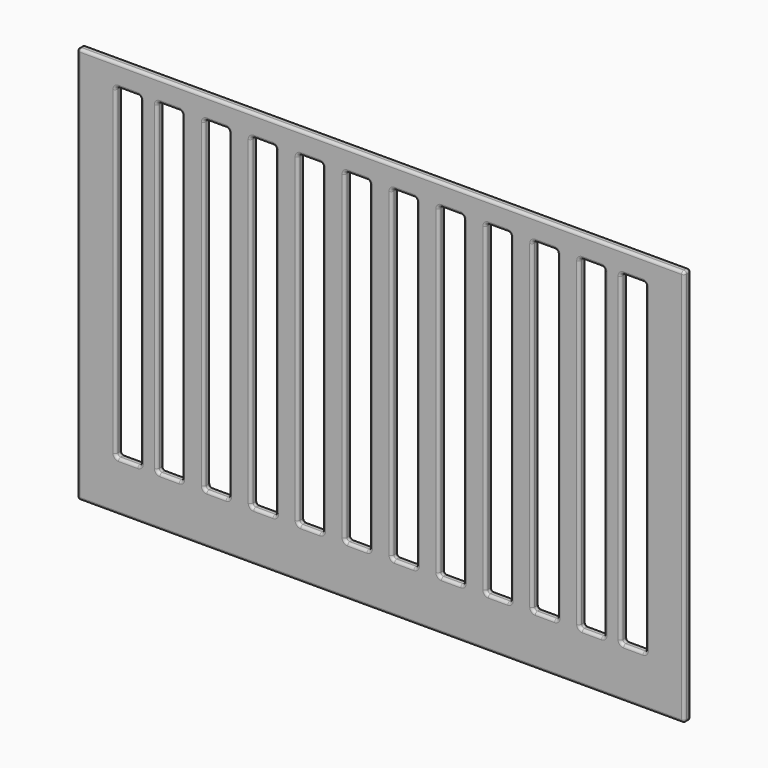
from build123d import *

# Parameters (mm, degrees)
F0_W     = 1397
F0_H     = 914.4
F1_DEPTH = 9.525
F2_W     = 57.15
F2_H     = 749.3
F3_DEPTH = 19.051
F4_F1_R  = 6.35
F4_F2_R  = 6.35
F4_F3_R  = 6.35


with BuildPart() as f1:
    # F0 (on Front) → F1 (new body, symmetric)
    with BuildSketch(Plane.XZ):
        Rectangle(F0_W, F0_H)
    extrude(amount=F1_DEPTH, both=True)

    # F2 (on face) → F3 (cut, through all)
    with BuildSketch(Plane.XZ.offset(9.525)):
        with Locations((-581.025, 31.75)):
            Rectangle(F2_W, F2_H)
        with Locations((-485.775, 31.75)):
            Rectangle(F2_W, F2_H)
        with Locations((-377.825, 31.75)):
            Rectangle(F2_W, F2_H)
        with Locations((-269.875, 31.75)):
            Rectangle(F2_W, F2_H)
        with Locations((-161.925, 31.75)):
            Rectangle(F2_W, F2_H)
        with Locations((-53.975, 31.75)):
            Rectangle(F2_W, F2_H)
        with Locations((53.975, 31.75)):
            Rectangle(F2_W, F2_H)
        with Locations((161.925, 31.75)):
            Rectangle(F2_W, F2_H)
        with Locations((269.875, 31.75)):
            Rectangle(F2_W, F2_H)
        with Locations((377.825, 31.75)):
            Rectangle(F2_W, F2_H)
        with Locations((485.775, 31.75)):
            Rectangle(F2_W, F2_H)
        with Locations((581.025, 31.75)):
            Rectangle(F2_W, F2_H)
    extrude(amount=-F3_DEPTH, mode=Mode.SUBTRACT)

    # F4: fillet of radius 6.35 on 135 edges, made by hand

    # F4_f1
    f4_f1_edges = [f1.edges().sort_by_distance(p)[0] for p in [
        (-82.55, 0, -342.9),
        (-82.55, 0, 406.4),
        (25.4, 0, -342.9),
        (25.4, 0, 406.4),
        (133.35, 0, -342.9),
        (133.35, 0, 406.4),
        (241.3, 0, -342.9),
        (241.3, 0, 406.4),
        (349.25, 0, -342.9),
        (349.25, 0, 406.4),
        (-190.5, 0, 406.4),
        (-298.45, 0, 406.4),
        (-241.3, 0, 406.4),
        (-406.4, 0, 406.4),
        (-349.25, 0, 406.4),
        (-514.35, 0, 406.4),
        (-457.2, 0, 406.4),
        (-609.6, 0, 406.4),
        (-552.45, 0, 406.4),
        (457.2, 0, -342.9),
        (457.2, 0, 406.4),
        (552.45, 0, -342.9),
        (552.45, 0, 406.4),
        (-552.45, 0, -342.9),
        (-609.6, 0, -342.9),
        (-457.2, 0, -342.9),
        (-514.35, 0, -342.9),
        (-349.25, 0, -342.9),
        (-406.4, 0, -342.9),
        (-241.3, 0, -342.9),
        (-298.45, 0, -342.9),
        (-133.35, 0, -342.9),
        (-190.5, 0, -342.9),
        (-25.4, 0, -342.9),
        (82.55, 0, -342.9),
        (190.5, 0, -342.9),
        (406.4, 0, -342.9),
        (514.35, 0, -342.9),
        (609.6, 0, -342.9),
        (609.6, 0, 406.4),
        (514.35, 0, 406.4),
        (406.4, 0, 406.4),
        (298.45, 0, 406.4),
        (298.45, 0, -342.9),
        (190.5, 0, 406.4),
        (82.55, 0, 406.4),
        (-25.4, 0, 406.4),
        (-133.35, 0, 406.4),
    ]]
    fillet(f4_f1_edges, radius=F4_F1_R)

    # F4_f2
    f4_f2_edges = [f1.edges().sort_by_distance(p)[0] for p in [
        (-698.5, -9.525, 0),
        (0, -9.525, 457.2),
        (0, 9.525, 457.2),
        (241.3, -9.525, 31.75),
        (241.3, 9.525, 31.75),
        (298.45, -9.525, 31.75),
        (698.5, 9.525, 0),
        (698.5, 0, 457.2),
        (698.5, -9.525, 0),
        (698.5, 0, -457.2),
        (-698.5, 0, 457.2),
        (-698.5, 9.525, 0),
        (-698.5, 0, -457.2),
        (0, 9.525, -457.2),
        (0, -9.525, -457.2),
        (298.45, 9.525, 31.75),
        (296.5901280605, 9.525, -341.0401280605),
        (296.5901280605, 9.525, 404.5401280605),
        (296.5901280605, -9.525, -341.0401280605),
        (296.5901280605, -9.525, 404.5401280605),
        (243.1598719395, 9.525, 404.5401280605),
        (243.1598719395, 9.525, -341.0401280605),
        (243.1598719395, -9.525, 404.5401280605),
        (243.1598719395, -9.525, -341.0401280605),
    ]]
    fillet(f4_f2_edges, radius=F4_F2_R)

    # F4_f3
    f4_f3_edges = [f1.edges().sort_by_distance(p)[0] for p in [
        (-609.6, -9.525, 31.75),
        (-609.6, 9.525, 31.75),
        (-552.45, -9.525, 31.75),
        (-514.35, -9.525, 31.75),
        (-514.35, 9.525, 31.75),
        (-457.2, -9.525, 31.75),
        (-406.4, -9.525, 31.75),
        (-406.4, 9.525, 31.75),
        (-349.25, -9.525, 31.75),
        (-298.45, -9.525, 31.75),
        (-298.45, 9.525, 31.75),
        (-241.3, -9.525, 31.75),
        (-269.875, -9.525, 406.4),
        (-377.825, -9.525, 406.4),
        (-485.775, -9.525, 406.4),
        (-581.025, -9.525, 406.4),
        (-161.925, -9.525, 406.4),
        (-190.5, -9.525, 31.75),
        (-190.5, 9.525, 31.75),
        (-133.35, -9.525, 31.75),
        (-82.55, -9.525, 31.75),
        (-82.55, 9.525, 31.75),
        (25.4, -9.525, 31.75),
        (25.4, 9.525, 31.75),
        (-25.4, -9.525, 31.75),
        (82.55, -9.525, 31.75),
        (133.35, -9.525, 31.75),
        (133.35, 9.525, 31.75),
        (190.5, -9.525, 31.75),
        (349.25, -9.525, 31.75),
        (349.25, 9.525, 31.75),
        (-269.875, 9.525, 406.4),
        (-377.825, 9.525, 406.4),
        (-485.775, 9.525, 406.4),
        (-581.025, 9.525, 406.4),
        (457.2, -9.525, 31.75),
        (457.2, 9.525, 31.75),
        (552.45, -9.525, 31.75),
        (552.45, 9.525, 31.75),
        (-581.025, -9.525, -342.9),
        (-581.025, 9.525, -342.9),
        (-485.775, -9.525, -342.9),
        (-485.775, 9.525, -342.9),
        (-377.825, -9.525, -342.9),
        (-377.825, 9.525, -342.9),
        (-269.875, -9.525, -342.9),
        (-269.875, 9.525, -342.9),
        (-161.925, -9.525, -342.9),
        (-161.925, 9.525, -342.9),
        (-53.975, -9.525, -342.9),
        (-53.975, 9.525, -342.9),
        (53.975, -9.525, -342.9),
        (53.975, 9.525, -342.9),
        (161.925, -9.525, -342.9),
        (161.925, 9.525, -342.9),
        (377.825, -9.525, -342.9),
        (377.825, 9.525, -342.9),
        (485.775, -9.525, -342.9),
        (485.775, 9.525, -342.9),
        (581.025, -9.525, -342.9),
        (581.025, 9.525, -342.9),
        (581.025, -9.525, 406.4),
        (581.025, 9.525, 406.4),
        (514.35, -9.525, 31.75),
        (514.35, 9.525, 31.75),
        (406.4, -9.525, 31.75),
        (406.4, 9.525, 31.75),
        (190.5, 9.525, 31.75),
        (82.55, 9.525, 31.75),
        (-25.4, 9.525, 31.75),
        (-133.35, 9.525, 31.75),
        (-135.2098719395, 9.525, -341.0401280605),
        (-135.2098719395, 9.525, 404.5401280605),
        (-27.2598719395, 9.525, -341.0401280605),
        (-27.2598719395, 9.525, 404.5401280605),
        (80.6901280605, 9.525, -341.0401280605),
        (80.6901280605, 9.525, 404.5401280605),
        (188.6401280605, 9.525, -341.0401280605),
        (188.6401280605, 9.525, 404.5401280605),
        (404.5401280605, 9.525, -341.0401280605),
        (404.5401280605, 9.525, 404.5401280605),
        (404.5401280605, -9.525, -341.0401280605),
        (404.5401280605, -9.525, 404.5401280605),
        (512.4901280605, 9.525, -341.0401280605),
        (512.4901280605, 9.525, 404.5401280605),
        (512.4901280605, -9.525, -341.0401280605),
        (512.4901280605, -9.525, 404.5401280605),
        (607.7401280605, 9.525, 404.5401280605),
        (554.3098719395, 9.525, 404.5401280605),
        (607.7401280605, -9.525, 404.5401280605),
        (554.3098719395, -9.525, 404.5401280605),
        (554.3098719395, 9.525, -341.0401280605),
        (607.7401280605, 9.525, -341.0401280605),
        (554.3098719395, -9.525, -341.0401280605),
        (607.7401280605, -9.525, -341.0401280605),
        (459.0598719395, 9.525, -341.0401280605),
        (459.0598719395, -9.525, -341.0401280605),
        (351.1098719395, 9.525, -341.0401280605),
        (351.1098719395, -9.525, -341.0401280605),
        (135.2098719395, 9.525, -341.0401280605),
        (135.2098719395, -9.525, -341.0401280605),
        (188.6401280605, -9.525, -341.0401280605),
        (27.2598719395, 9.525, -341.0401280605),
        (27.2598719395, -9.525, -341.0401280605),
        (80.6901280605, -9.525, -341.0401280605),
        (-80.6901280605, 9.525, -341.0401280605),
        (-80.6901280605, -9.525, -341.0401280605),
        (-27.2598719395, -9.525, -341.0401280605),
        (-188.6401280605, 9.525, -341.0401280605),
        (-188.6401280605, -9.525, -341.0401280605),
        (-135.2098719395, -9.525, -341.0401280605),
        (-296.5901280605, 9.525, -341.0401280605),
        (-243.1598719395, 9.525, -341.0401280605),
        (-296.5901280605, -9.525, -341.0401280605),
        (-243.1598719395, -9.525, -341.0401280605),
        (-404.5401280605, 9.525, -341.0401280605),
        (-351.1098719395, 9.525, -341.0401280605),
        (-404.5401280605, -9.525, -341.0401280605),
        (-351.1098719395, -9.525, -341.0401280605),
        (-512.4901280605, 9.525, -341.0401280605),
        (-459.0598719395, 9.525, -341.0401280605),
        (-512.4901280605, -9.525, -341.0401280605),
        (-459.0598719395, -9.525, -341.0401280605),
        (-607.7401280605, 9.525, -341.0401280605),
        (-554.3098719395, 9.525, -341.0401280605),
        (-607.7401280605, -9.525, -341.0401280605),
        (-554.3098719395, -9.525, -341.0401280605),
        (459.0598719395, 9.525, 404.5401280605),
        (459.0598719395, -9.525, 404.5401280605),
        (-554.3098719395, 9.525, 404.5401280605),
        (-607.7401280605, 9.525, 404.5401280605),
        (-459.0598719395, 9.525, 404.5401280605),
        (-512.4901280605, 9.525, 404.5401280605),
        (-351.1098719395, 9.525, 404.5401280605),
        (-404.5401280605, 9.525, 404.5401280605),
        (-243.1598719395, 9.525, 404.5401280605),
        (-296.5901280605, 9.525, 404.5401280605),
        (351.1098719395, 9.525, 404.5401280605),
        (351.1098719395, -9.525, 404.5401280605),
        (188.6401280605, -9.525, 404.5401280605),
        (135.2098719395, 9.525, 404.5401280605),
        (135.2098719395, -9.525, 404.5401280605),
        (80.6901280605, -9.525, 404.5401280605),
        (-27.2598719395, -9.525, 404.5401280605),
        (27.2598719395, 9.525, 404.5401280605),
        (27.2598719395, -9.525, 404.5401280605),
        (-80.6901280605, 9.525, 404.5401280605),
        (-80.6901280605, -9.525, 404.5401280605),
        (-135.2098719395, -9.525, 404.5401280605),
        (-188.6401280605, 9.525, 404.5401280605),
        (-188.6401280605, -9.525, 404.5401280605),
        (-554.3098719395, -9.525, 404.5401280605),
        (-607.7401280605, -9.525, 404.5401280605),
        (-459.0598719395, -9.525, 404.5401280605),
        (-512.4901280605, -9.525, 404.5401280605),
        (-351.1098719395, -9.525, 404.5401280605),
        (-404.5401280605, -9.525, 404.5401280605),
        (-243.1598719395, -9.525, 404.5401280605),
        (-296.5901280605, -9.525, 404.5401280605),
    ]]
    fillet(f4_f3_edges, radius=F4_F3_R)


solid = f1.part
